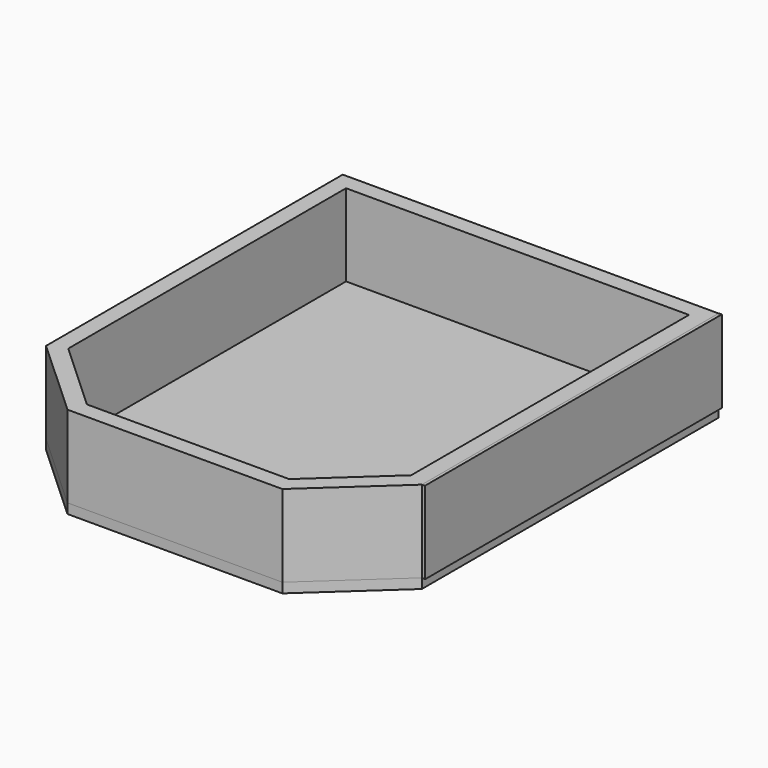
from build123d import *

# Parameters (mm, degrees)
F1_DEPTH  = 76.2
F2_DEPTH  = 635
F2_FACE_W = 2870.2
F2_FACE_H = 635
F3_DEPTH  = 25.4
F3_TAPER  = -3


with BuildPart() as f1:
    # F0 (on Top) → F1 (new body)
    with BuildSketch(Plane.XY):
        Polygon((2908.3, 0), (0, 0), (0, -2870.2), (622.3, -3441.7), (2286, -3441.7), (2908.3, -2870.2), align=None)
        Polygon((671.7684459615, -3314.7), (127, -2814.4024475864), (127, -127), (2781.3, -127), (2781.3, -2814.4024475864), (2236.5315540385, -3314.7), align=None, mode=Mode.SUBTRACT)
        Polygon((127, -127), (127, -2814.4024475864), (671.7684459615, -3314.7), (2236.5315540385, -3314.7), (2781.3, -2814.4024475864), (2781.3, -127), align=None)
    extrude(amount=-F1_DEPTH)


with BuildPart() as f2:
    # F0 (on Top) → F2 (new body)
    with BuildSketch(Plane.XY):
        Polygon((2908.3, 0), (0, 0), (0, -2870.2), (622.3, -3441.7), (2286, -3441.7), (2908.3, -2870.2), align=None)
        Polygon((671.7684459615, -3314.7), (127, -2814.4024475864), (127, -127), (2781.3, -127), (2781.3, -2814.4024475864), (2236.5315540385, -3314.7), align=None, mode=Mode.SUBTRACT)
    extrude(amount=F2_DEPTH)

    # F2_face (on face) → F3 (join)
    with BuildSketch(Plane(origin=(2908.3, -1435.1, 317.5), x_dir=(0, 1, 0), z_dir=(1, 0, 0))):
        Rectangle(F2_FACE_W, F2_FACE_H)
    extrude(amount=F3_DEPTH, taper=F3_TAPER)


solid = Compound([f1.part, f2.part])
